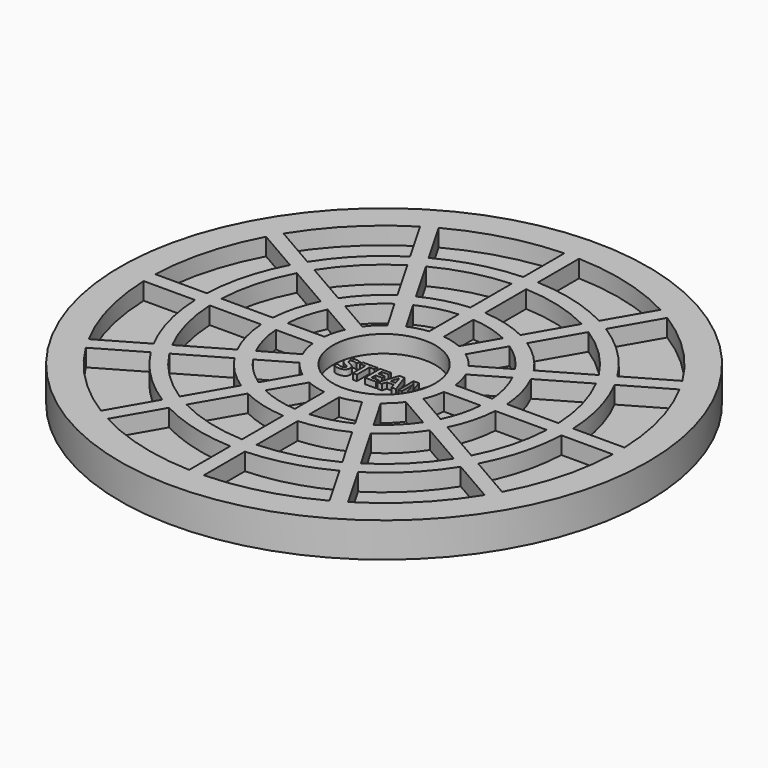
from build123d import *

# Parameters (mm, degrees)
F0_R          = 22.86
F1_DEPTH      = 3
F2_R          = 4.445
F3_DEPTH      = 1.5
F4_R          = 8.89
F4_R_2        = 5.715
F5_DEPTH      = 1.5
F6_R          = 14.605
F6_R_2        = 10.16
F7_DEPTH      = 1.5
F8_R          = 20.32
F8_R_2        = 15.875
F9_DEPTH      = 1.5
F10_W         = 1.27
F10_H         = 16.51
F10_W_2       = 16.51
F10_H_2       = 1.27
F11_DEPTH     = 1.5
F12_TEXT_SIZE = 2.310732054
F13_DEPTH     = 0.5


# Not quite as in the source:
# - Text() gives the source's letters only with a copy of the font that has no kerning and outlines rounded to 1/6400 em; it was checked with that copy


with BuildPart() as f1:
    # F0 (on Top) → F1 (new body)
    with BuildSketch(Plane.XY):
        Circle(F0_R)
    extrude(amount=F1_DEPTH)

    # F2 (on face) → F3 (cut)
    with BuildSketch(Plane.XY.offset(3)):
        Circle(F2_R)
    extrude(amount=-F3_DEPTH, mode=Mode.SUBTRACT)

    # F4 (on face) → F5 (cut)
    with BuildSketch(Plane.XY.offset(3)):
        Circle(F4_R)
        Circle(F4_R_2, mode=Mode.SUBTRACT)
    extrude(amount=-F5_DEPTH, mode=Mode.SUBTRACT)

    # F6 (on face) → F7 (cut)
    with BuildSketch(Plane.XY.offset(3)):
        Circle(F6_R)
        Circle(F6_R_2, mode=Mode.SUBTRACT)
    extrude(amount=-F7_DEPTH, mode=Mode.SUBTRACT)

    # F8 (on face) → F9 (cut)
    with BuildSketch(Plane.XY.offset(3)):
        Circle(F8_R)
        Circle(F8_R_2, mode=Mode.SUBTRACT)
    extrude(amount=-F9_DEPTH, mode=Mode.SUBTRACT)

    # F10 (on face) → F11 (join)
    with BuildSketch(Plane.XY.offset(1.5)):
        with Locations((0, -13.081)):
            Rectangle(F10_W, F10_H)
        Polygon((11.2179261314, -18.1600180151), (2.9629261314, -3.8619385987), (1.8630738686, -4.4969385987), (10.1180738686, -18.7950180151), align=None)
        Polygon((18.7950180151, -10.1180738686), (4.4969385987, -1.8630738686), (3.8619385987, -2.9629261314), (18.1600180151, -11.2179261314), align=None)
        with Locations((13.081, 0)):
            Rectangle(F10_W_2, F10_H_2)
        Polygon((18.1600180151, 11.2179261314), (3.8619385987, 2.9629261314), (4.4969385987, 1.8630738686), (18.7950180151, 10.1180738686), align=None)
        Polygon((10.1180738686, 18.7950180151), (1.8630738686, 4.4969385987), (2.9629261314, 3.8619385987), (11.2179261314, 18.1600180151), align=None)
        with Locations((0, 13.081)):
            Rectangle(F10_W, F10_H)
        Polygon((-11.2179261314, 18.1600180151), (-2.9629261314, 3.8619385987), (-1.8630738686, 4.4969385987), (-10.1180738686, 18.7950180151), align=None)
        Polygon((-18.7950180151, 10.1180738686), (-4.4969385987, 1.8630738686), (-3.8619385987, 2.9629261314), (-18.1600180151, 11.2179261314), align=None)
        with Locations((-13.081, 0)):
            Rectangle(F10_W_2, F10_H_2)
        Polygon((-18.1600180151, -11.2179261314), (-3.8619385987, -2.9629261314), (-4.4969385987, -1.8630738686), (-18.7950180151, -10.1180738686), align=None)
        Polygon((-10.1180738686, -18.7950180151), (-1.8630738686, -4.4969385987), (-2.9629261314, -3.8619385987), (-11.2179261314, -18.1600180151), align=None)
    extrude(amount=F11_DEPTH)

    # F12 (on face) → F13 (join)
    with BuildSketch(Plane.XY.offset(1.5)):
        with Locations((-3.81, -0.8318635394)):
            Text('STEAM', F12_TEXT_SIZE, font='Open Sans', font_style=FontStyle.BOLD, text_align=(TextAlign.LEFT, TextAlign.BOTTOM))
    extrude(amount=F13_DEPTH)


solid = f1.part
